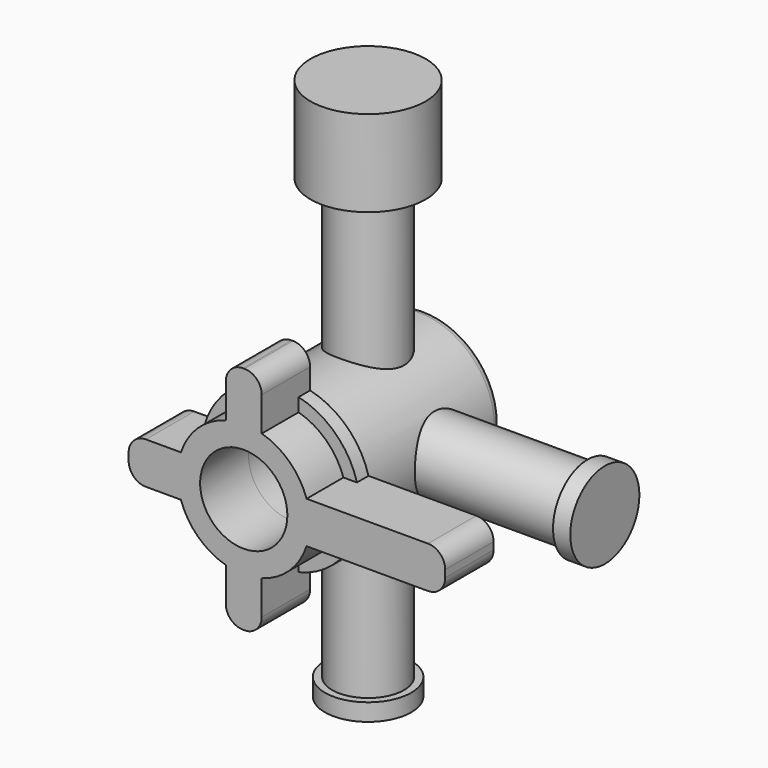
from build123d import *

# Parameters (mm, degrees)
F0_R      = 6.6675
F1_DEPTH  = 14.732
F2_R      = 3.175
F3_DEPTH  = 19.3675
F4_R      = 3.175
F5_DEPTH  = 19.3675
F6_R      = 0.762
F7_R      = 5.08
F8_DEPTH  = 7.62
F9_R      = 3.81
F10_DEPTH = 1.524
F11_R     = 3.81
F12_DEPTH = 1.524
F13_R     = 6.985
F14_DEPTH = 1.27
F15_R     = 5.842
F15_R_2   = 3.81
F16_DEPTH = 4.064
F17_W     = 3.175
F17_H     = 20.32
F18_DEPTH = 5.334
F19_W     = 27.94
F19_H     = 3.683
F20_DEPTH = 5.334
F21_R     = 3.8489929185
F22_DEPTH = 12.7
F23_R     = 1.524


with BuildPart() as f1:
    # F0 (on Front) → F1 (new body)
    with BuildSketch(Plane.XZ):
        Circle(F0_R)
    extrude(amount=F1_DEPTH)

    # F2 (on Top) → F3 (join, symmetric)
    with BuildSketch(Plane.XY):
        with Locations((0, -6.35)):
            Circle(F2_R)
    extrude(amount=F3_DEPTH, both=True)

    # F4 (on Right) → F5 (join)
    with BuildSketch(Plane.YZ):
        with Locations((-6.35, 0)):
            Circle(F4_R)
    extrude(amount=F5_DEPTH)

    # F6
    f6_edges = [f1.edges().sort_by_distance(p)[0] for p in [
        (-6.6675, 0, 0),
    ]]
    fillet(f6_edges, radius=F6_R)

    # F7 (on face) → F8 (join)
    with BuildSketch(Plane.XY.offset(19.3675)):
        with Locations((0, -6.35)):
            Circle(F7_R)
    extrude(amount=F8_DEPTH)

    # F9 (on face) → F10 (join)
    with BuildSketch(Plane.YZ.offset(19.3675)):
        with Locations((-6.35, 0)):
            Circle(F9_R)
    extrude(amount=F10_DEPTH)

    # F11 (on face) → F12 (join)
    with BuildSketch(Plane(origin=(0, 0, -19.3675), x_dir=(1, 0, 0), z_dir=(0, 0, -1))):
        with Locations((0, 6.35)):
            Circle(F11_R)
    extrude(amount=F12_DEPTH)


with BuildPart() as f14:
    # F13 (on face) → F14 (new body)
    with BuildSketch(Plane.XZ.offset(14.732)):
        Circle(F13_R)
    extrude(amount=F14_DEPTH)

    # F15 (on face) → F16 (join)
    with BuildSketch(Plane.XZ.offset(16.002)):
        Circle(F15_R)
        Circle(F15_R_2, mode=Mode.SUBTRACT)
    extrude(amount=F16_DEPTH)

    # F17 (on face) → F18 (join, through all)
    with BuildSketch(Plane(origin=(0, -14.732, 0), x_dir=(-1, 0, 0), z_dir=(0, 1, 0))):
        Rectangle(F17_W, F17_H)
    extrude(amount=-F18_DEPTH)

    # F19 (on face) → F20 (join, through all)
    with BuildSketch(Plane(origin=(0, -14.732, 0), x_dir=(-1, 0, 0), z_dir=(0, 1, 0))):
        with Locations((-3.81, 0)):
            Rectangle(F19_W, F19_H)
    extrude(amount=-F20_DEPTH)


with BuildPart() as f22_tool:
    # F21 (on face) → F22 (new body)
    with BuildSketch(Plane.XZ.offset(20.066)):
        Circle(F21_R)
    extrude(amount=-F22_DEPTH)


with BuildPart() as f1_1:
    add(f1.part)

    # F22: cut by f22_tool
    add(f22_tool.part, mode=Mode.SUBTRACT)


with BuildPart() as f14_1:
    add(f14.part)

    # F22: cut by f22_tool
    add(f22_tool.part, mode=Mode.SUBTRACT)

    # F23
    f23_edges = [f14_1.edges().sort_by_distance(p)[0] for p in [
        (17.78, -17.399, -1.8415),
        (17.78, -17.399, 1.8415),
        (1.5875, -17.399, 10.16),
        (-1.5875, -17.399, 10.16),
        (-10.16, -17.399, 1.8415),
        (-10.16, -17.399, -1.8415),
        (-1.5875, -17.399, -10.16),
        (1.5875, -17.399, -10.16),
    ]]
    fillet(f23_edges, radius=F23_R)


solid = Compound([f1_1.part, f14_1.part])
